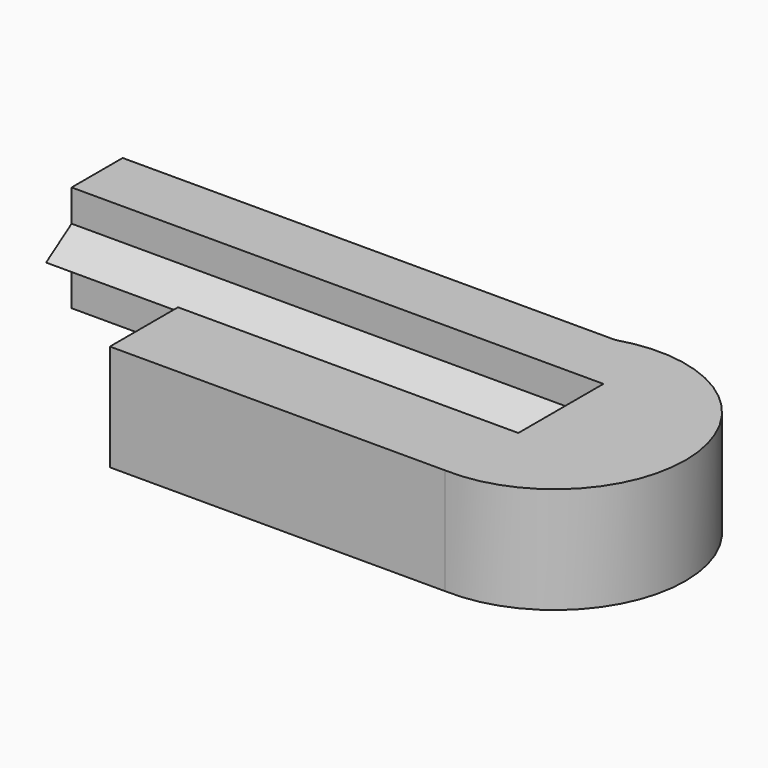
from build123d import *

# Parameters (mm, degrees)
F1_DEPTH = 1.27
F3_DEPTH = 12.7
F6_DEPTH = 1.778


with BuildPart() as f1:
    # F0 (on Top) → F1 (new body, symmetric)
    with BuildSketch(Plane.XY):
        with BuildLine():
            Line((0, 1.524), (0, 0))
            Line((0, 0), (12.7, 0))
            Line((12.7, 0), (12.7, -2.54))
            Line((12.7, -2.54), (4.572, -2.54))
            Line((4.572, -2.54), (4.572, -4.572))
            Line((4.572, -4.572), (12.5717104354, -4.572))
            ThreePointArc((12.5717104354, -4.572), (15.7940682602, -1.0438103752), (11.7644204026, 1.524))
            Line((11.7644204026, 1.524), (0, 1.524))
        make_face()
    extrude(amount=F1_DEPTH, both=True)

    # F2 (on face) → F3 (join, through all)
    with BuildSketch(Plane(origin=(0, 0, 0), x_dir=(0, -1, 0), z_dir=(-1, 0, 0))):
        Polygon((0.762, 0), (0, 0.508), (0, -0.508), align=None)
    extrude(amount=-F3_DEPTH)

    # F5 (on face) → F6 (join)
    with BuildSketch(Plane(origin=(0, 0, 0), x_dir=(0, -1, 0), z_dir=(-1, 0, 0))):
        Polygon((-4.064, -1.27), (-1.524, -1.27), (-1.524, 1.27), align=None)
    extrude(amount=-F6_DEPTH)


with BuildPart() as f7_1:
    # F7: copy of F1
    add(f1.part)


solid = f1.part
